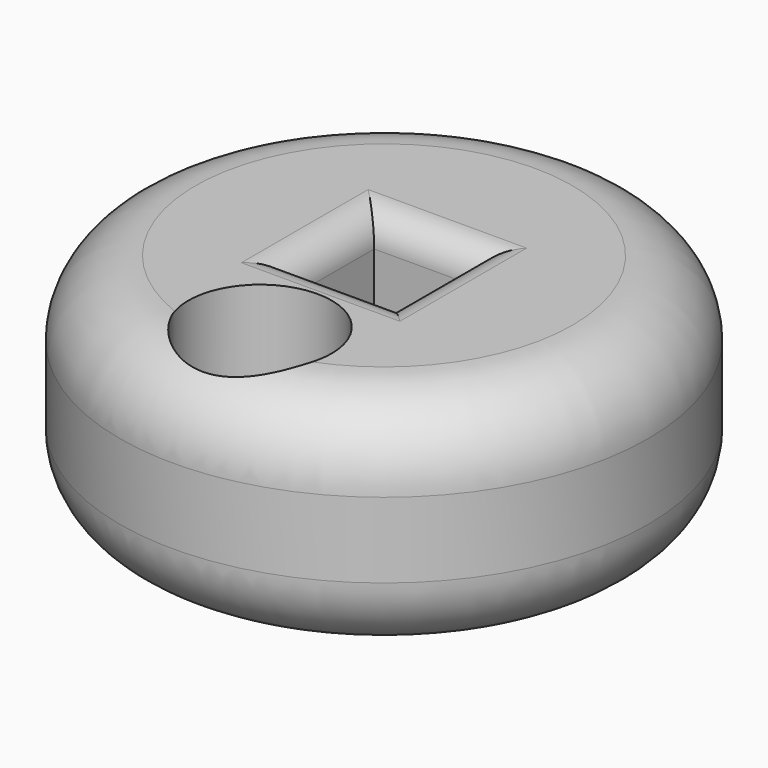
from build123d import *

# Parameters (mm, degrees)
F0_R     = 17.5
F0_R_2   = 4.75
F0_W     = 6.5
F0_H     = 6.5
F1_DEPTH = 15
F3_R     = 2


# Not quite as in the source:
# - a fillet or chamfer that OpenCascade refuses, or shapes differently, is made with other operations: its cross-section is extruded or revolved along the edge and cut away or added
# - a feature names something its author has since deleted; it is built from what else it names


with BuildPart() as f1:
    # F0 (on Top) → F1 (new body)
    with BuildSketch(Plane.XY):
        Circle(F0_R)
        with Locations((0, -10.2685028687)):
            Circle(F0_R_2, mode=Mode.SUBTRACT)
        Rectangle(F0_W, F0_H, mode=Mode.SUBTRACT)
    extrude(amount=F1_DEPTH)

    # F2: fillet of radius 5 on 2 edges, made by hand

    # F2_s1 → F2_t2 (revolve, cut)
    with BuildSketch(Plane.XZ):
        with BuildLine():
            ThreePointArc((17.5, 10), (16.0355339059, 13.5355339059), (12.5, 15))
            Line((12.5, 15), (17.5, 15))
            Line((17.5, 15), (17.5, 10))
        make_face()
    revolve(axis=Axis((0, 0, 15), (0, 0, 1)), mode=Mode.SUBTRACT)

    # F2_s3 → F2_t4 (revolve, cut)
    with BuildSketch(Plane.XZ):
        with BuildLine():
            ThreePointArc((17.5, 5), (16.0355339059, 1.4644660941), (12.5, 0))
            Line((12.5, 0), (17.5, 0))
            Line((17.5, 0), (17.5, 5))
        make_face()
    revolve(axis=Axis((0, 0, 0), (0, 0, 1)), mode=Mode.SUBTRACT)

    # F3
    f3_edges = [f1.edges().sort_by_distance(p)[0] for p in [
        (-3.25, 0, 15),
        (0, -3.25, 15),
        (0, 3.25, 15),
        (3.25, 0, 15),
        (-3.25, 0, 0),
        (0, -3.25, 0),
        (3.25, 0, 0),
        (0, 3.25, 0),
    ]]
    fillet(f3_edges, radius=F3_R)


solid = f1.part
